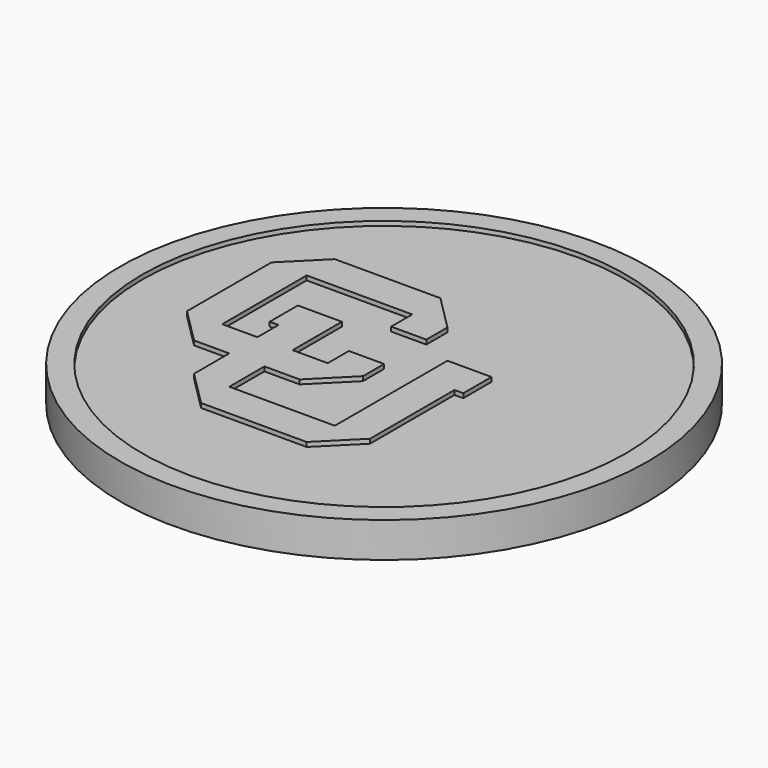
from build123d import *

# Parameters (mm, degrees)
F0_R           = 38.1
F1_DEPTH       = 3.81
F3_R           = 38.1
F3_R_2         = 34.925
F4_DEPTH       = 0.635
F6_R           = 38.1
F6_R_2         = 34.925
F6_TEXT_SIZE   = 17.8470659274
F6_TEXT_SIZE_2 = 17.2504907943
F7_DEPTH       = 0.635


# Not quite as in the source:
# - Text() gives the source's letters only with a copy of the font that has no kerning and outlines rounded to 1/6400 em; it was checked with that copy


with BuildPart() as f1:
    # F0 (on Top) → F1 (new body)
    with BuildSketch(Plane.XY):
        Circle(F0_R)
    extrude(amount=F1_DEPTH)

    # F3 (on face) → F4 (join)
    with BuildSketch(Plane.XY.offset(3.81)):
        Circle(F3_R)
        Circle(F3_R_2, mode=Mode.SUBTRACT)
        Polygon((0, -3.81), (0, 0), (-5.08, 0), (-5.08, -3.81), (-10.16, -3.81), (-10.16, 5.08), (-16.51, 5.08), (-16.51, 0), (-15.24, 0), (-15.24, -3.81), (-20.32, -3.81), (-20.32, 11.43), (-5.08, 11.43), (-5.08, 7.62), (0, 7.62), (0, 11.43), (-5.08, 16.51), (-20.32, 16.51), (-25.4, 11.43), (-25.4, -3.81), (-20.32, -8.89), (-15.24, -8.89), (-15.24, -15.24), (-10.16, -20.32), (5.08, -20.32), (10.16, -15.24), (10.16, 0), (11.43, 0), (11.43, 5.08), (5.08, 5.08), (5.08, -15.24), (-10.16, -15.24), (-10.16, -8.89), (-5.08, -8.89), align=None)
    extrude(amount=F4_DEPTH)

    # F6 (on face) → F7 (join)
    with BuildSketch(Plane(origin=(0, 0, 0), x_dir=(1, 0, 0), z_dir=(0, 0, -1))):
        Circle(F6_R)
        Circle(F6_R_2, mode=Mode.SUBTRACT)
        with Locations((-25.4, -17.9298874677)):
            Text('Aguas', F6_TEXT_SIZE, font='Open Sans', text_align=(TextAlign.LEFT, TextAlign.BOTTOM))
        with Locations((-25.4, 5.08)):
            Text('Daniel', F6_TEXT_SIZE_2, font='Open Sans', text_align=(TextAlign.LEFT, TextAlign.BOTTOM))
    extrude(amount=F7_DEPTH)


solid = f1.part
